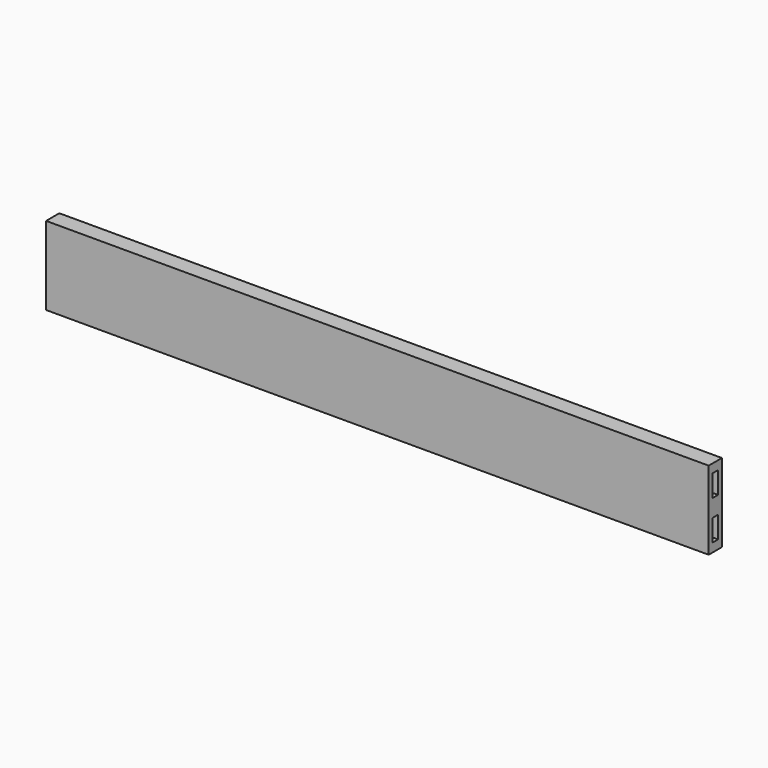
from build123d import *

# Parameters (mm, degrees)
F0_W     = 760
F0_H     = 90
F1_DEPTH = 19
F2_W     = 8
F2_H     = 25
F3_DEPTH = 25


# Not quite as in the source:
# - a pattern or mirror of a feature is missing from the dataset's text; its kind, count and spacing are read off the source's solid


with BuildPart() as f1:
    # F0 (on Front) → F1 (new body)
    with BuildSketch(Plane.XZ):
        Rectangle(F0_W, F0_H)
    extrude(amount=F1_DEPTH)

    # F2 (on face) → F3 (cut)
    with BuildSketch(Plane(origin=(-380, 0, 0), x_dir=(0, -1, 0), z_dir=(-1, 0, 0))):
        with Locations((9.5, 22.5)):
            Rectangle(F2_W, F2_H)
        with Locations((9.5, -22.5)):
            Rectangle(F2_W, F2_H)
    f3 = extrude(amount=-F3_DEPTH, mode=Mode.SUBTRACT)

    # F3_copies: F3 across plane
    add(f3.mirror(Plane(origin=(0, 0, 0), x_dir=(0, 0, 1), z_dir=(1, 0, 0))), mode=Mode.SUBTRACT)


solid = f1.part
